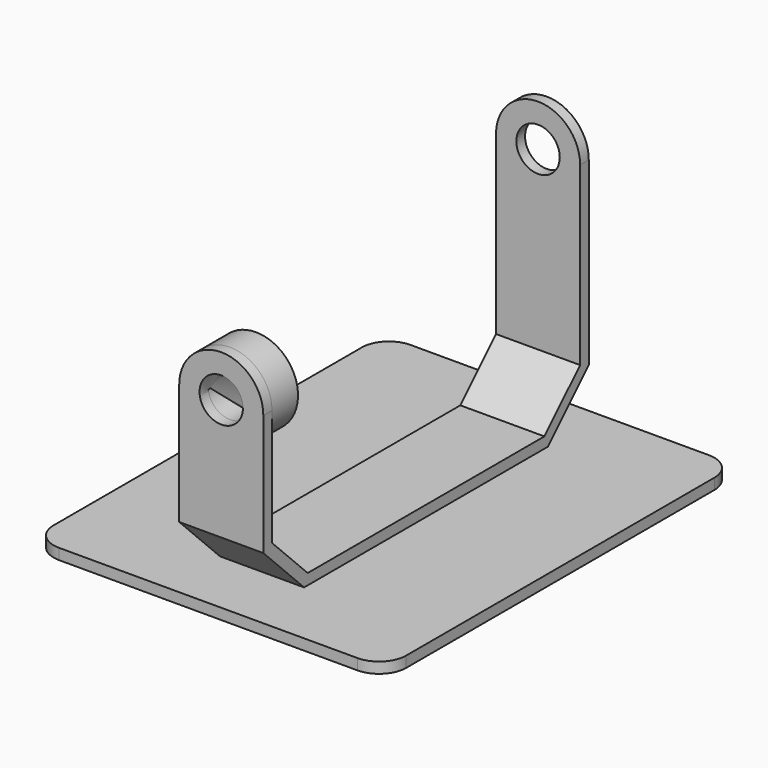
from build123d import *

# Parameters (mm, degrees)
F1_DEPTH  = 7.75
F3_DEPTH  = 2
F4_R      = 4
F5_DEPTH  = 2
F6_R      = 4
F7_DEPTH  = 6
F9_DEPTH  = 2
F11_DEPTH = 2
F12_W     = 65
F12_H     = 81
F12_W_2   = 15.5
F12_H_2   = 56.2027688981
F13_DEPTH = 2
F14_R     = 5


with BuildPart() as f1:
    # F0 (on Right) → F1 (new body, symmetric)
    with BuildSketch(Plane.YZ):
        Polygon((0, 0), (0, 21.5), (-2, 21.5), (-2, -0.8284271247), (7.398615551, -10.2270426757), (56.688359309, -10.2270426757), (63.601384449, -10.2270426757), (73, -0.8284271247), (73, 32.5), (71, 32.5), (71, 0), (62.7729573243, -8.2270426757), (8.2270426757, -8.2270426757), align=None)
    extrude(amount=F1_DEPTH, both=True)

    # F2 (on face) → F3 (join)
    with BuildSketch(Plane.XZ.offset(2)):
        with BuildLine():
            Line((-7.75, 21.5), (7.75, 21.5))
            ThreePointArc((7.75, 21.5), (0, 29.25), (-7.75, 21.5))
        make_face()
    extrude(amount=-F3_DEPTH)

    # F4 (on face) → F5 (cut)
    with BuildSketch(Plane.XZ.offset(2)):
        with Locations((0, 21.5)):
            Circle(F4_R)
    extrude(amount=-F5_DEPTH, mode=Mode.SUBTRACT)

    # F6 (on face) → F7 (join)
    with BuildSketch(Plane(origin=(0, 0, 0), x_dir=(-1, 0, 0), z_dir=(0, 1, 0))):
        with BuildLine():
            ThreePointArc((-7.75, 21.5), (0, 13.75), (7.75, 21.5))
            ThreePointArc((7.75, 21.5), (0, 29.25), (-7.75, 21.5))
        make_face()
        with Locations((0, 21.5)):
            Circle(F6_R, mode=Mode.SUBTRACT)
    extrude(amount=F7_DEPTH)

    # F8 (on face) → F9 (join)
    with BuildSketch(Plane(origin=(0, 73, 0), x_dir=(-1, 0, 0), z_dir=(0, 1, 0))):
        with BuildLine():
            Line((-7.75, 32.5), (7.75, 32.5))
            ThreePointArc((7.75, 32.5), (0, 40.25), (-7.75, 32.5))
        make_face()
    extrude(amount=-F9_DEPTH)

    # F10 (on face) → F11 (cut)
    with BuildSketch(Plane(origin=(0, 73, 0), x_dir=(-1, 0, 0), z_dir=(0, 1, 0))):
        with BuildLine():
            Line((-4, 32.5), (4, 32.5))
            ThreePointArc((4, 32.5), (0, 36.5), (-4, 32.5))
        make_face()
        with BuildLine():
            ThreePointArc((-4, 32.5), (0, 28.5), (4, 32.5))
            Line((4, 32.5), (-4, 32.5))
        make_face()
    extrude(amount=-F11_DEPTH, mode=Mode.SUBTRACT)

    # F12 (on face) → F13 (join)
    with BuildSketch(Plane(origin=(0, 0, -10.2270426757), x_dir=(1, 0, 0), z_dir=(0, 0, -1))):
        with Locations((0, -35.5)):
            Rectangle(F12_W, F12_H)
        with Locations((0, -35.5)):
            Rectangle(F12_W_2, F12_H_2, mode=Mode.SUBTRACT)
        with Locations((0, -35.5)):
            Rectangle(F12_W_2, F12_H_2)
    extrude(amount=F13_DEPTH)

    # F14
    f14_edges = [f1.edges().sort_by_distance(p)[0] for p in [
        (32.5, -5, -11.227043),
        (-32.5, -5, -11.227043),
        (-32.5, 76, -11.227043),
        (32.5, 76, -11.227043),
    ]]
    fillet(f14_edges, radius=F14_R)


solid = f1.part
